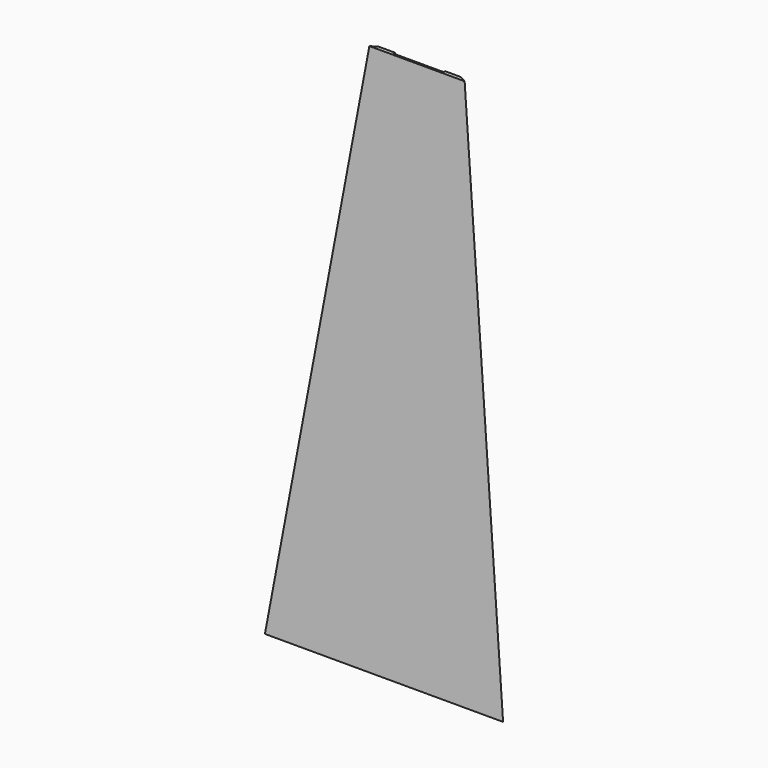
from build123d import *

# Parameters (mm, degrees)
F7_R      = 960.2431856589
F8_DEPTH  = 635.5163904251
F12_R     = 870.2287794889
F13_DEPTH = 25
F14_R     = 892.9375722879
F15_DEPTH = 25
F19_REACH = 785.9273977736


with BuildPart() as f5:
    # F3 (on Top) → F5 section 0
    with BuildSketch(Plane.XY):
        Polygon((-375, -216.5063509461), (375, -216.5063509461), (0, 433.0127018922), align=None)
    # F4 (on line) → F5 section 1
    with BuildSketch(Plane.XY.offset(1650)):
        Polygon((-150, -86.6025403784), (150, -86.6025403784), (0, 173.2050807569), align=None)
    loft()

    # F7 (on face) → F8 (cut, through all)
    with BuildSketch(Plane(origin=(0, -203.2096543416, 15.9986111776), x_dir=(1, 0, 0), z_dir=(0, -0.9969151597, 0.078486714))):
        with Locations((0, 812.9688501358)):
            Circle(F7_R)
    extrude(amount=-F8_DEPTH, mode=Mode.SUBTRACT)

    # F12 (on face) → F13 (cut)
    with BuildSketch(Plane(origin=(0, 0, 0), x_dir=(0.8660254038, -0.5, 0), z_dir=(-0.5, -0.8660254038, 0))):
        with Locations((304.0688931942, 817.2121047974)):
            Circle(F12_R)
    extrude(amount=-F13_DEPTH, mode=Mode.SUBTRACT)

    # F14 (on face) → F15 (cut)
    with BuildSketch(Plane(origin=(0, 0, 0), x_dir=(-0.8660254038, -0.5, 0), z_dir=(-0.5, 0.8660254038, 0))):
        with Locations((291.6465699673, 811.1194968224)):
            Circle(F14_R)
    extrude(amount=F15_DEPTH, mode=Mode.SUBTRACT)

    f19_end = Plane(origin=(0, -155.5781982198, 697.4454188962), x_dir=(0, 0.078486714, 0.9969151597), z_dir=(0, 0.9969151597, -0.078486714))
    # F17 (on Front) → F19 (cut, up to a plane its end follows)
    with BuildSketch(Plane.XZ):
        Polygon((80.7874383415, 1638), (79.1510747051, 1650), (-79.1510747051, 1650), (-80.7874383415, 1638), align=None)
        Polygon((-94.7891388542, 1420), (110.5147110688, 1420), (108.8783474324, 1432), (-93.1527752178, 1432), align=None)
        Polygon((237.6056201597, 488), (235.9692565233, 500), (-239.4393885352, 500), (-241.0757521715, 488), align=None)
        Polygon((-286.2211157241, 70), (294.6056201597, 70), (292.9692565233, 82), (-284.5847520878, 82), align=None)
    f19_long = extrude(amount=F19_REACH, mode=Mode.PRIVATE)
    add(split(f19_long, bisect_by=f19_end, keep=Keep.TOP, mode=Mode.PRIVATE), mode=Mode.SUBTRACT)


solid = f5.part
